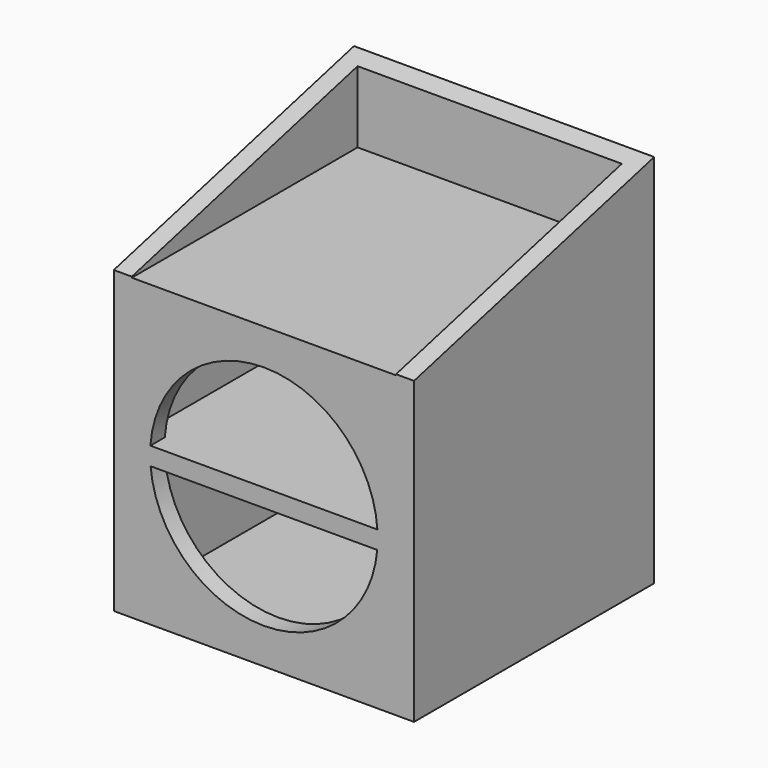
from build123d import *

# Parameters (mm, degrees)
F1_DEPTH = 100
F2_T     = -12
F3_W     = 176
F3_H     = 12
F4_DEPTH = 188
F6_DEPTH = 12


with BuildPart() as f1:
    # F0 (on Right) → F1 (new body, symmetric)
    with BuildSketch(Plane.YZ):
        Polygon((-124.4957186917, 75.0704253932), (-124.4957186917, -124.9295746068), (75.5042813083, -124.9295746068), (75.5042813083, 125.0704253932), align=None)
    extrude(amount=F1_DEPTH, both=True)

    # F2
    f2_openings = [f1.faces().sort_by_distance(p)[0] for p in [
        (0, -124.495719, -24.929575),
        (0, -24.495719, 100.070425),
    ]]
    offset(amount=F2_T, openings=f2_openings)

    # F3 (on face) → F4 (join)
    with BuildSketch(Plane.XZ.offset(-63.5042813083)):
        with Locations((0, -26.0345488787)):
            Rectangle(F3_W, F3_H)
        with Locations((0, 68.4323040247)):
            Rectangle(F3_W, F3_H)
    extrude(amount=F4_DEPTH)

    # F5 (on face) → F6 (join)
    with BuildSketch(Plane.XZ.offset(124.4957186917)):
        Polygon((100, -124.9295746068), (100, 75.0704253932), (88, 75.0704253932), (88, 74.4323040247), (-88, 74.4323040247), (-88, 75.0704253932), (-100, 75.0704253932), (-100, -124.9295746068), align=None)
        Polygon((88, -112.9295746068), (-88, -112.9295746068), (-88, -32.0345488787), (-88, -20.0345488787), (-88, 62.4323040247), (88, 62.4323040247), (88, -20.0345488787), (88, -32.0345488787), align=None, mode=Mode.SUBTRACT)
        with BuildLine():
            Line((-88, 62.4323040247), (-88, -20.0345488787))
            Line((-88, -20.0345488787), (-75.6174618507, -20.0345488787))
            ThreePointArc((-75.6174618507, -20.0345488787), (0, 50.4918066225), (75.6174618507, -20.0345488787))
            Line((75.6174618507, -20.0345488787), (88, -20.0345488787))
            Line((88, -20.0345488787), (88, 62.4323040247))
            Line((88, 62.4323040247), (-88, 62.4323040247))
        make_face()
        with BuildLine():
            Line((-88, -32.0345488787), (-88, -112.9295746068))
            Line((-88, -112.9295746068), (88, -112.9295746068))
            Line((88, -112.9295746068), (88, -32.0345488787))
            Line((88, -32.0345488787), (75.5022996144, -32.0345488787))
            ThreePointArc((75.5022996144, -32.0345488787), (0, -101.1106302402), (-75.5022996144, -32.0345488787))
            Line((-75.5022996144, -32.0345488787), (-88, -32.0345488787))
        make_face()
    extrude(amount=-F6_DEPTH)


solid = f1.part
